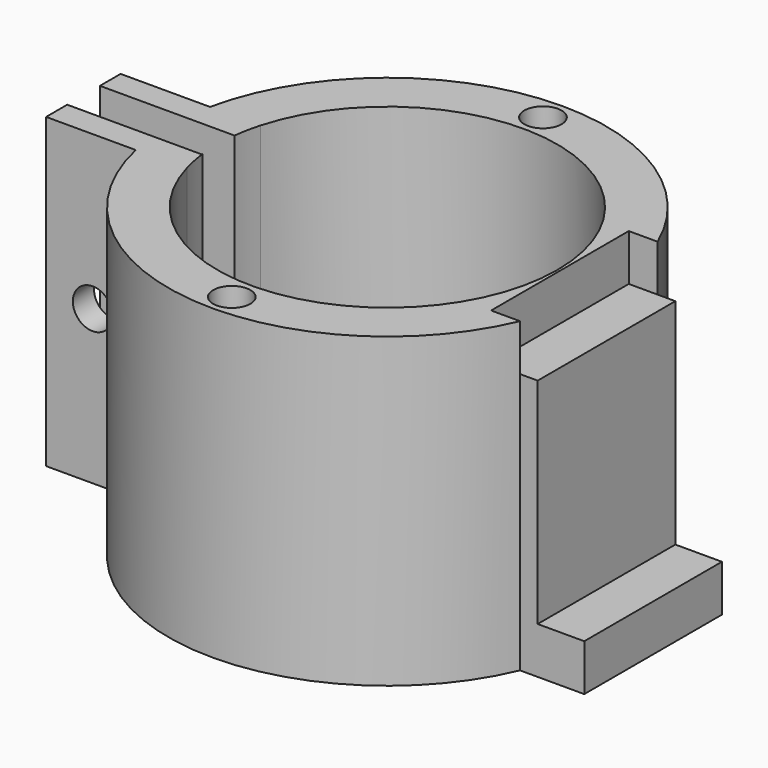
from build123d import *

# Parameters (mm, degrees)
F1_DEPTH  = 33
F3_W      = 1.8808413297
F3_H      = 18.471846357
F4_DEPTH  = 33
F5_R      = 2
F6_DEPTH  = 3
F7_W      = 18.471846357
F7_H      = 5
F8_DEPTH  = 5
F9_DEPTH  = 5
F2_R      = 2.125
F10_DEPTH = 25


# Not quite as in the source:
# - a feature names something its author has since deleted; it is built from what else it names


with BuildPart() as f1:
    # F0 (on Top) → F1 (new body)
    with BuildSketch(Plane.XY):
        with BuildLine():
            ThreePointArc((-23.401635828, 2.1478921234), (-23.2315061267, 3.5421918479), (-22.9783775489, 4.9238364331))
            Line((-22.9783775489, 4.9238364331), (-32.5732277849, 4.9238364331))
            Line((-32.5732277849, 4.9238364331), (-32.5732277849, 2.1478921234))
            Line((-32.5732277849, 2.1478921234), (-23.401635828, 2.1478921234))
        make_face()
        with BuildLine():
            Line((-32.5732277849, -5.0761635669), (-22.9452078535, -5.0761635669))
            ThreePointArc((-22.9452078535, -5.0761635669), (-23.2124017724, -3.6652972535), (-23.3929275249, -2.2407458164))
            Line((-23.3929275249, -2.2407458164), (-32.5732277849, -2.2407458164))
            Line((-32.5732277849, -2.2407458164), (-32.5732277849, -5.0761635669))
        make_face()
        with BuildLine():
            ThreePointArc((-22.9452078535, -5.0761635669), (2.55319559, -23.3608902287), (23.5, 0))
            ThreePointArc((23.5, 0), (2.4756946097, 23.3692305436), (-22.9783775489, 4.9238364331))
            Line((-22.9783775489, 4.9238364331), (-17.5732277849, 4.9238364331))
            ThreePointArc((-17.5732277849, 4.9238364331), (2.4850646798, 18.080015308), (18.25, 0))
            ThreePointArc((18.25, 0), (2.4850646798, -18.080015308), (-17.5732277849, -4.9238364331))
            Line((-17.5732277849, -4.9238364331), (-17.5732277849, -5.0761635669))
            Line((-17.5732277849, -5.0761635669), (-22.9452078535, -5.0761635669))
        make_face()
        with BuildLine():
            Line((-17.5732277849, 4.9238364331), (-22.9783775489, 4.9238364331))
            ThreePointArc((-22.9783775489, 4.9238364331), (-23.2315061267, 3.5421918479), (-23.401635828, 2.1478921234))
            Line((-23.401635828, 2.1478921234), (-18.1231636153, 2.1478921234))
            ThreePointArc((-18.1231636153, 2.1478921234), (-17.9020824613, 3.5465396584), (-17.5732277849, 4.9238364331))
        make_face()
        with BuildLine():
            ThreePointArc((-23.3929275249, -2.2407458164), (-23.2124017724, -3.6652972535), (-22.9452078535, -5.0761635669))
            Line((-22.9452078535, -5.0761635669), (-17.5732277849, -5.0761635669))
            Line((-17.5732277849, -5.0761635669), (-17.5732277849, -4.9238364331))
            ThreePointArc((-17.5732277849, -4.9238364331), (-17.9020824613, -3.5465396584), (-18.1231636153, -2.1478921234))
            Line((-18.1231636153, -2.1478921234), (-18.1231636153, -2.2407458164))
            Line((-18.1231636153, -2.2407458164), (-23.3929275249, -2.2407458164))
        make_face()
    extrude(amount=F1_DEPTH)

    # F3 (on Top) → F4 (join)
    with BuildSketch(Plane.XY):
        with Locations((22.5681019947, 0.0180900097)):
            Rectangle(F3_W, F3_H)
    extrude(amount=F4_DEPTH)

    # F5 (on face) → F6 (cut)
    with BuildSketch(Plane.XY.offset(33)):
        with Locations((0, 20.875)):
            Circle(F5_R)
        with Locations((0, -20.875)):
            Circle(F5_R)
    extrude(amount=-F6_DEPTH, mode=Mode.SUBTRACT)

    # F7 (on face) → F8 (cut)
    with BuildSketch(Plane.YZ.offset(23.5085226595)):
        with Locations((0.0180900097, 30.5)):
            Rectangle(F7_W, F7_H)
    extrude(amount=-F8_DEPTH, mode=Mode.SUBTRACT)

    # F7 (on face) → F9 (join)
    with BuildSketch(Plane.YZ.offset(23.5085226595)):
        with Locations((0.0180900097, 2.5)):
            Rectangle(F7_W, F7_H)
    extrude(amount=F9_DEPTH)

    # F2 (on face) → F10 (cut)
    with BuildSketch(Plane.XZ.offset(5.0761635669)):
        with Locations((-27.5732277849, 16.5)):
            Circle(F2_R)
    extrude(amount=-F10_DEPTH, mode=Mode.SUBTRACT)


solid = f1.part
